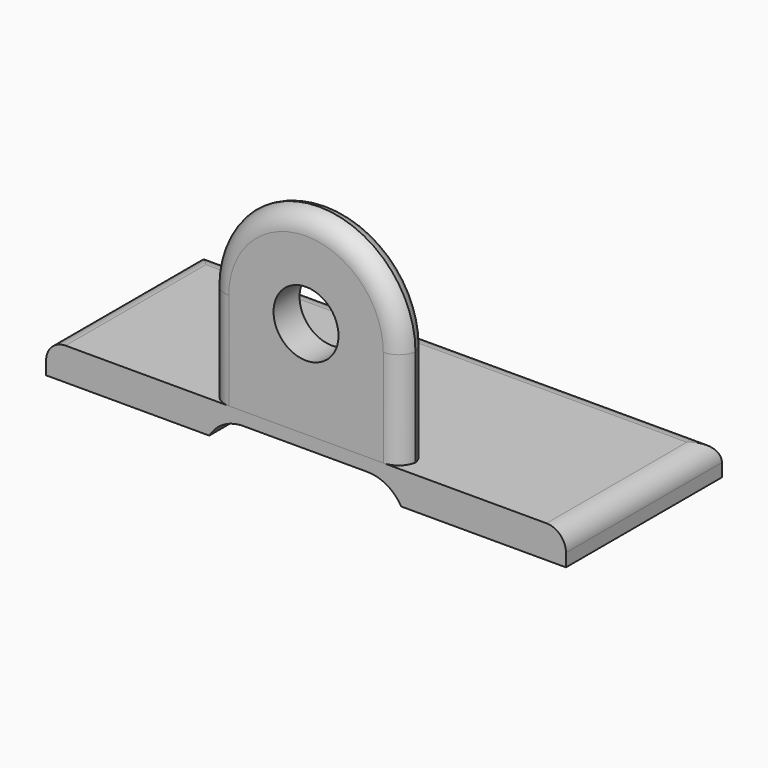
from build123d import *

# Parameters (mm, degrees)
F0_W          = 80
F0_H          = 30
F1_DEPTH      = 5
F2_R          = 5
F3_DEPTH      = 5
F4_W          = 29.5208403841
F4_H          = 3
F5_DEPTH      = 30.001
F6_T1_DEPTH   = 30
F7_T1_DEPTH   = 45
F7_T3_DEPTH   = 95
F7_2_T1_DEPTH = 22.5
F7_2_T4_ANGLE = 180
F7_2_T6_ANGLE = 180


# Not quite as in the source:
# - a fillet or chamfer that OpenCascade refuses, or shapes differently, is made with other operations: its cross-section is extruded or revolved along the edge and cut away or added


with BuildPart() as f1:
    # F0 (on Top) → F1 (new body)
    with BuildSketch(Plane.XY):
        Rectangle(F0_W, F0_H)
    extrude(amount=F1_DEPTH)

    # F4 (on face) → F5 (cut, through all)
    with BuildSketch(Plane.XZ.offset(15)):
        with Locations((-0.1258742996, 1.5)):
            Rectangle(F4_W, F4_H)
    extrude(amount=-F5_DEPTH, mode=Mode.SUBTRACT)

    # F6: fillet of radius 6 on 2 edges, made by hand

    # F6_s2 → F6_t1 (join)
    with BuildSketch(Plane.XZ.offset(-15)):
        with BuildLine():
            ThreePointArc((-14.8862944916, 0), (-12.6901420689, 2.1961524227), (-9.6901420689, 3))
            Line((-9.6901420689, 3), (-14.8862944916, 3))
            Line((-14.8862944916, 3), (-14.8862944916, 0))
        make_face()
        with BuildLine():
            ThreePointArc((9.4383934698, 3), (12.4383934698, 2.1961524227), (14.6345458925, 0))
            Line((14.6345458925, 0), (14.6345458925, 3))
            Line((14.6345458925, 3), (9.4383934698, 3))
        make_face()
    extrude(amount=F6_T1_DEPTH)

    # F7: fillet of radius 3 on 3 edges, made by hand

    # F7_s2 → F7_t1 (cut)
    with BuildSketch(Plane.XZ.offset(-22.5)):
        with BuildLine():
            ThreePointArc((40, 2), (39.1213203436, 4.1213203436), (37, 5))
            Line((37, 5), (40, 5))
            Line((40, 5), (40, 2))
        make_face()
        with BuildLine():
            ThreePointArc((-37, 5), (-39.1213203436, 4.1213203436), (-40, 2))
            Line((-40, 2), (-40, 5))
            Line((-40, 5), (-37, 5))
        make_face()
    extrude(amount=F7_T1_DEPTH, mode=Mode.SUBTRACT)

    # F7_s4 → F7_t3 (cut)
    with BuildSketch(Plane.YZ.offset(-47.5)):
        with BuildLine():
            ThreePointArc((12, 5), (14.1213203436, 4.1213203436), (15, 2))
            Line((15, 2), (15, 5))
            Line((15, 5), (12, 5))
        make_face()
    extrude(amount=F7_T3_DEPTH, mode=Mode.SUBTRACT)


with BuildPart() as f3:
    # F2 (on face) → F3 (new body)
    with BuildSketch(Plane.XZ.offset(15)):
        with BuildLine():
            Line((-14.8862944916, 20), (-14.8862944916, 5))
            Line((-14.8862944916, 5), (14.8862944916, 5))
            Line((14.8862944916, 5), (14.8862944916, 20))
            ThreePointArc((14.8862944916, 20), (0, 34.8862944916), (-14.8862944916, 20))
        make_face()
        with Locations((0, 20)):
            Circle(F2_R, mode=Mode.SUBTRACT)
    extrude(amount=-F3_DEPTH)

    # F7#2: fillet of radius 3 on 6 edges, made by hand

    # F7_2_s2 → F7_2_t1 (cut)
    with BuildSketch(Plane.XY.offset(-2.5)):
        with BuildLine():
            ThreePointArc((14.8862944916, -12), (14.0076148351, -14.1213203436), (11.8862944916, -15))
            Line((11.8862944916, -15), (14.8862944916, -15))
            Line((14.8862944916, -15), (14.8862944916, -12))
        make_face()
        with BuildLine():
            ThreePointArc((14.8862944916, -13), (14.0076148351, -10.8786796564), (11.8862944916, -10))
            Line((11.8862944916, -10), (14.8862944916, -10))
            Line((14.8862944916, -10), (14.8862944916, -13))
        make_face()
        with BuildLine():
            ThreePointArc((-14.8862944916, -12), (-14.0076148351, -14.1213203436), (-11.8862944916, -15))
            Line((-11.8862944916, -15), (-14.8862944916, -15))
            Line((-14.8862944916, -15), (-14.8862944916, -12))
        make_face()
        with BuildLine():
            ThreePointArc((-14.8862944916, -13), (-14.0076148351, -10.8786796564), (-11.8862944916, -10))
            Line((-11.8862944916, -10), (-14.8862944916, -10))
            Line((-14.8862944916, -10), (-14.8862944916, -13))
        make_face()
    extrude(amount=F7_2_T1_DEPTH, mode=Mode.SUBTRACT)

    # F7_2_s3 → F7_2_t4 (revolve, cut)
    with BuildSketch(Plane.XY.offset(20)):
        with BuildLine():
            ThreePointArc((14.8862944916, -12), (14.0076148351, -14.1213203436), (11.8862944916, -15))
            Line((11.8862944916, -15), (14.8862944916, -15))
            Line((14.8862944916, -15), (14.8862944916, -12))
        make_face()
    revolve(axis=Axis((0, -15, 20), (0, -1, 0)), revolution_arc=F7_2_T4_ANGLE, mode=Mode.SUBTRACT)

    # F7_2_s5 → F7_2_t6 (revolve, cut)
    with BuildSketch(Plane.XY.offset(20)):
        with BuildLine():
            ThreePointArc((14.8862944916, -13), (14.0076148351, -10.8786796564), (11.8862944916, -10))
            Line((11.8862944916, -10), (14.8862944916, -10))
            Line((14.8862944916, -10), (14.8862944916, -13))
        make_face()
    revolve(axis=Axis((0, -10, 20), (0, -1, 0)), revolution_arc=F7_2_T6_ANGLE, mode=Mode.SUBTRACT)


solid = Compound([f1.part, f3.part])
